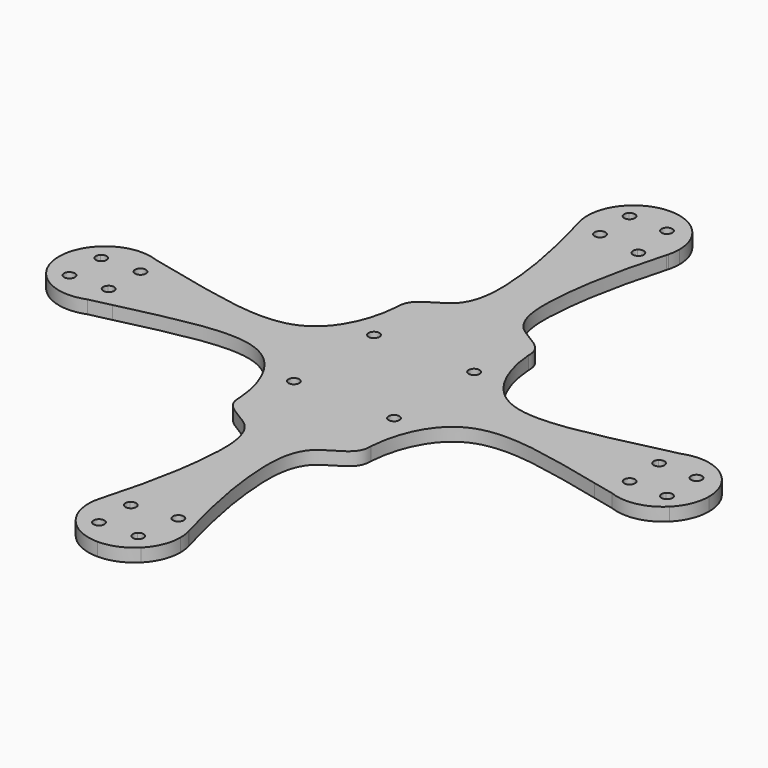
from build123d import *

# Parameters (mm, degrees)
F0_W     = 20
F0_H     = 30
F0_R     = 1.65
F1_DEPTH = 4


with BuildPart() as f1:
    # F0 (on Top) → F1 (new body)
    with BuildSketch(Plane.XY):
        with BuildLine():
            ThreePointArc((9.8994949366, 104.8994949366), (5.3575680531, 107.9343134552), (0, 109))
            Line((0, 109), (0, 95))
            Line((0, 95), (4.4901280605, 99.4901280605))
            ThreePointArc((4.4901280605, 99.4901280605), (4.4901280605, 101.8235804385), (6.8235804385, 101.8235804385))
            Line((6.8235804385, 101.8235804385), (9.8994949366, 104.8994949366))
        make_face()
        with BuildLine():
            Line((0, 95), (0, 109))
            ThreePointArc((0, 109), (-5.3575680531, 107.9343134552), (-9.8994949366, 104.8994949366))
            Line((-9.8994949366, 104.8994949366), (-7.177133829, 102.177133829))
            ThreePointArc((-7.177133829, 102.177133829), (-5.3789799767, 102.5348088687), (-4.3604076401, 101.0104076401))
            ThreePointArc((-4.3604076401, 101.0104076401), (-4.4860064114, 100.3789799767), (-4.8436814511, 99.8436814511))
            Line((-4.8436814511, 99.8436814511), (0, 95))
        make_face()
        with BuildLine():
            Line((6.2578950135, 88.7421049865), (0, 95))
            Line((0, 95), (0, 81))
            ThreePointArc((0, 81), (5.3575680531, 82.0656865448), (9.8994949366, 85.1005050634))
            Line((9.8994949366, 85.1005050634), (8.5913473914, 86.4086526086))
            ThreePointArc((8.5913473914, 86.4086526086), (6.2578950135, 86.4086526086), (6.2578950135, 88.7421049865))
        make_face()
        with BuildLine():
            Line((0, 81), (0, 95))
            Line((0, 95), (-4.4901280605, 90.5098719395))
            ThreePointArc((-4.4901280605, 90.5098719395), (-4.1324530208, 89.9745734139), (-4.0068542495, 89.3431457505))
            ThreePointArc((-4.0068542495, 89.3431457505), (-5.0254265861, 87.8187445219), (-6.8235804385, 88.1764195615))
            Line((-6.8235804385, 88.1764195615), (-9.8994949366, 85.1005050634))
            ThreePointArc((-9.8994949366, 85.1005050634), (-5.3575680531, 82.0656865448), (0, 81))
        make_face()
        with BuildLine():
            Line((-4.4901280605, 90.5098719395), (0, 95))
            Line((0, 95), (-4.8436814511, 99.8436814511))
            ThreePointArc((-4.8436814511, 99.8436814511), (-7.177133829, 99.8436814511), (-7.177133829, 102.177133829))
            Line((-7.177133829, 102.177133829), (-9.8994949366, 104.8994949366))
            ThreePointArc((-9.8994949366, 104.8994949366), (-13.5184120598, 98.6404031894), (-13.5319969205, 91.4104235148))
            add(Edge.make_bspline(
                [(-13.3797592699, 90.8790726917), (-13.4302497753, 91.0559438951), (-13.4809959841, 91.2330606372), (-13.5319969205, 91.4104235148)],
                knots=[0.9938840637, 0.9938840637, 0.9938840637, 0.9938840637, 1, 1, 1, 1], degree=3))
            ThreePointArc((-13.3797592699, 90.8790726917), (-11.9928678831, 87.7770421614), (-9.8994949366, 85.1005050634))
            Line((-9.8994949366, 85.1005050634), (-6.8235804385, 88.1764195615))
            ThreePointArc((-6.8235804385, 88.1764195615), (-6.8235804385, 90.5098719395), (-4.4901280605, 90.5098719395))
        make_face()
        with BuildLine():
            Line((4.4901280605, 99.4901280605), (0, 95))
            Line((0, 95), (6.2578950135, 88.7421049865))
            ThreePointArc((6.2578950135, 88.7421049865), (8.0560488659, 89.0997800262), (9.0746212025, 87.5753787975))
            ThreePointArc((9.0746212025, 87.5753787975), (8.9490224311, 86.9439511341), (8.5913473914, 86.4086526086))
            Line((8.5913473914, 86.4086526086), (9.8994949366, 85.1005050634))
            ThreePointArc((9.8994949366, 85.1005050634), (11.9928678831, 87.7770421614), (13.3797592699, 90.8790726917))
            add(Edge.make_bspline(
                [(13.3797592699, 90.8790726917), (13.4302497753, 91.0559438951), (13.4809959841, 91.2330606372), (13.5319969205, 91.4104235148)],
                knots=[0.9938840637, 0.9938840637, 0.9938840637, 0.9938840637, 1, 1, 1, 1], degree=3))
            ThreePointArc((13.5319969205, 91.4104235148), (13.8825062018, 93.1900216697), (14, 95))
            ThreePointArc((14, 95), (12.9343134552, 100.3575680531), (9.8994949366, 104.8994949366))
            Line((9.8994949366, 104.8994949366), (6.8235804385, 101.8235804385))
            ThreePointArc((6.8235804385, 101.8235804385), (7.1812554781, 101.2882819129), (7.3068542495, 100.6568542495))
            ThreePointArc((7.3068542495, 100.6568542495), (6.2882819129, 99.1324530208), (4.4901280605, 99.4901280605))
        make_face()
        with BuildLine():
            ThreePointArc((9.8994949366, 85.1005050634), (5.3575680531, 82.0656865448), (0, 81))
            Line((0, 81), (0, 30))
            Line((0, 30), (20, 30))
            add(Edge.make_bspline(
                [(20, 30), (20.2946353761, 35.7326359325), (6.8531098255, 37.7432494173), (6.0119172559, 59.8139246806), (9.9463832068, 78.8517548594), (13.3797592699, 90.8790726917)],
                knots=[0, 0, 0, 0, 0.2669632141, 0.5779977645, 0.9938840637, 0.9938840637, 0.9938840637, 0.9938840637], degree=3))
            ThreePointArc((13.3797592699, 90.8790726917), (11.9928678831, 87.7770421614), (9.8994949366, 85.1005050634))
        make_face()
        with BuildLine():
            Line((0, 30), (0, 81))
            ThreePointArc((0, 81), (-5.3575680531, 82.0656865448), (-9.8994949366, 85.1005050634))
            ThreePointArc((-9.8994949366, 85.1005050634), (-11.9928678831, 87.7770421614), (-13.3797592699, 90.8790726917))
            add(Edge.make_bspline(
                [(-20, 30), (-20.2946353761, 35.7326359325), (-6.8531098255, 37.7432494173), (-6.0119172559, 59.8139246806), (-9.9463832068, 78.8517548594), (-13.3797592699, 90.8790726917)],
                knots=[0, 0, 0, 0, 0.2669632141, 0.5779977645, 0.9938840637, 0.9938840637, 0.9938840637, 0.9938840637], degree=3))
            Line((-20, 30), (0, 30))
        make_face()
        with BuildLine():
            add(Edge.make_bspline(
                [(-13.3797592699, 90.8790726917), (-13.4302497753, 91.0559438951), (-13.4809959841, 91.2330606372), (-13.5319969205, 91.4104235148)],
                knots=[0.9938840637, 0.9938840637, 0.9938840637, 0.9938840637, 1, 1, 1, 1], degree=3))
            ThreePointArc((-13.5319969205, 91.4104235148), (-13.4585006125, 91.1439967242), (-13.3797592699, 90.8790726917))
        make_face()
        with Locations((10, 15)):
            Rectangle(F0_W, F0_H)
        with Locations((15.25, 15.25)):
            Circle(F0_R, mode=Mode.SUBTRACT)
        with Locations((-10, 15)):
            Rectangle(F0_W, F0_H)
        with Locations((-15.25, 15.25)):
            Circle(F0_R, mode=Mode.SUBTRACT)
        with BuildLine():
            ThreePointArc((13.3797592699, 90.8790726917), (13.4585006125, 91.1439967242), (13.5319969205, 91.4104235148))
            add(Edge.make_bspline(
                [(13.3797592699, 90.8790726917), (13.4302497753, 91.0559438951), (13.4809959841, 91.2330606372), (13.5319969205, 91.4104235148)],
                knots=[0.9938840637, 0.9938840637, 0.9938840637, 0.9938840637, 1, 1, 1, 1], degree=3))
        make_face()
        with Locations((10, -15)):
            Rectangle(F0_W, F0_H)
        with Locations((15.25, -15.25)):
            Circle(F0_R, mode=Mode.SUBTRACT)
        with Locations((-10, -15)):
            Rectangle(F0_W, F0_H)
        with Locations((-15.25, -15.25)):
            Circle(F0_R, mode=Mode.SUBTRACT)
        with BuildLine():
            add(Edge.make_bspline(
                [(20, 30), (20.6434332622, 21.0878026995), (29.0666934116, 0.5854139886), (55.4305406227, 7.3872741481), (73.4306914551, 11.5693085449)],
                knots=[0, 0, 0, 0, 0.4161099486, 0.9383621207, 0.9383621207, 0.9383621207, 0.9383621207], degree=3))
            Line((20, 30), (20, 0))
            Line((20, 0), (71, 0))
            ThreePointArc((71, 0), (72.0656865448, 5.3575680531), (75.1005050634, 9.8994949366))
            Line((75.1005050634, 9.8994949366), (73.4306914551, 11.5693085449))
        make_face()
        with BuildLine():
            Line((-20, 0), (-20, 30))
            add(Edge.make_bspline(
                [(-20, 30), (-20.6434332622, 21.0878026995), (-29.0666934116, 0.5854139886), (-55.4305406227, 7.3872741481), (-73.4306914551, 11.5693085449)],
                knots=[0, 0, 0, 0, 0.4161099486, 0.9383621207, 0.9383621207, 0.9383621207, 0.9383621207], degree=3))
            Line((-73.4306914551, 11.5693085449), (-75.1005050634, 9.8994949366))
            ThreePointArc((-75.1005050634, 9.8994949366), (-72.0656865448, 5.3575680531), (-71, 0))
            Line((-71, 0), (-20, 0))
        make_face()
        with BuildLine():
            Line((20, -30), (0, -30))
            Line((0, -30), (0, -81))
            ThreePointArc((0, -81), (5.3575680531, -82.0656865448), (9.8994949366, -85.1005050634))
            ThreePointArc((9.8994949366, -85.1005050634), (11.9928678831, -87.7770421614), (13.3797592699, -90.8790726917))
            add(Edge.make_bspline(
                [(20, -30), (20.2946353761, -35.7326359325), (6.8531098255, -37.7432494173), (6.0119172559, -59.8139246806), (9.9463832068, -78.8517548594), (13.3797592699, -90.8790726917)],
                knots=[0, 0, 0, 0, 0.2669632141, 0.5779977645, 0.9938840637, 0.9938840637, 0.9938840637, 0.9938840637], degree=3))
        make_face()
        with BuildLine():
            Line((0, -81), (0, -30))
            Line((0, -30), (-20, -30))
            add(Edge.make_bspline(
                [(-20, -30), (-20.2946353761, -35.7326359325), (-6.8531098255, -37.7432494173), (-6.0119172559, -59.8139246806), (-9.9463832068, -78.8517548594), (-13.3797592699, -90.8790726917)],
                knots=[0, 0, 0, 0, 0.2669632141, 0.5779977645, 0.9938840637, 0.9938840637, 0.9938840637, 0.9938840637], degree=3))
            ThreePointArc((-13.3797592699, -90.8790726917), (-11.9928678831, -87.7770421614), (-9.8994949366, -85.1005050634))
            ThreePointArc((-9.8994949366, -85.1005050634), (-5.3575680531, -82.0656865448), (0, -81))
        make_face()
        with BuildLine():
            Line((-20, -30), (-20, 0))
            Line((-20, 0), (-71, 0))
            ThreePointArc((-71, 0), (-72.0656865448, -5.3575680531), (-75.1005050634, -9.8994949366))
            Line((-75.1005050634, -9.8994949366), (-73.4306914551, -11.5693085449))
            add(Edge.make_bspline(
                [(-20, -30), (-20.6434332622, -21.0878026995), (-29.0666934116, -0.5854139886), (-55.4305406227, -7.3872741481), (-73.4306914551, -11.5693085449)],
                knots=[0, 0, 0, 0, 0.4161099486, 0.9383621207, 0.9383621207, 0.9383621207, 0.9383621207], degree=3))
        make_face()
        with BuildLine():
            Line((71, 0), (20, 0))
            Line((20, 0), (20, -30))
            add(Edge.make_bspline(
                [(20, -30), (20.6434332622, -21.0878026995), (29.0666934116, -0.5854139886), (55.4305406227, -7.3872741481), (73.4306914551, -11.5693085449)],
                knots=[0, 0, 0, 0, 0.4161099486, 0.9383621207, 0.9383621207, 0.9383621207, 0.9383621207], degree=3))
            Line((73.4306914551, -11.5693085449), (75.1005050634, -9.8994949366))
            ThreePointArc((75.1005050634, -9.8994949366), (72.0656865448, -5.3575680531), (71, 0))
        make_face()
        with BuildLine():
            add(Edge.make_bspline(
                [(73.4306914551, 11.5693085449), (75.5551270882, 12.0628856806), (77.7259083603, 12.5619846054), (79.9393690816, 13.0533526233)],
                knots=[0.9383621207, 0.9383621207, 0.9383621207, 0.9383621207, 1, 1, 1, 1], degree=3))
            Line((73.4306914551, 11.5693085449), (75.1005050634, 9.8994949366))
            ThreePointArc((75.1005050634, 9.8994949366), (77.3555218637, 11.7286808305), (79.9393690816, 13.0533526233))
        make_face()
        with BuildLine():
            Line((-75.1005050634, 9.8994949366), (-73.4306914551, 11.5693085449))
            add(Edge.make_bspline(
                [(-73.4306914551, 11.5693085449), (-75.5551270882, 12.0628856806), (-77.7259083603, 12.5619846054), (-79.9393690816, 13.0533526233)],
                knots=[0.9383621207, 0.9383621207, 0.9383621207, 0.9383621207, 1, 1, 1, 1], degree=3))
            ThreePointArc((-79.9393690816, 13.0533526233), (-77.3555218637, 11.7286808305), (-75.1005050634, 9.8994949366))
        make_face()
        with BuildLine():
            ThreePointArc((9.8994949366, -85.1005050634), (5.3575680531, -82.0656865448), (0, -81))
            Line((0, -81), (0, -95))
            Line((0, -95), (6.2578950135, -88.7421049865))
            ThreePointArc((6.2578950135, -88.7421049865), (6.2578950135, -86.4086526086), (8.5913473914, -86.4086526086))
            Line((8.5913473914, -86.4086526086), (9.8994949366, -85.1005050634))
        make_face()
        with BuildLine():
            Line((0, -95), (0, -81))
            ThreePointArc((0, -81), (-5.3575680531, -82.0656865448), (-9.8994949366, -85.1005050634))
            Line((-9.8994949366, -85.1005050634), (-6.8235804385, -88.1764195615))
            ThreePointArc((-6.8235804385, -88.1764195615), (-5.0254265861, -87.8187445219), (-4.0068542495, -89.3431457505))
            ThreePointArc((-4.0068542495, -89.3431457505), (-4.1324530208, -89.9745734139), (-4.4901280605, -90.5098719395))
            Line((-4.4901280605, -90.5098719395), (0, -95))
        make_face()
        with BuildLine():
            ThreePointArc((-75.1005050634, -9.8994949366), (-72.0656865448, -5.3575680531), (-71, 0))
            Line((-71, 0), (-85, 0))
            Line((-85, 0), (-80.5098719395, -4.4901280605))
            ThreePointArc((-80.5098719395, -4.4901280605), (-78.7117180871, -4.1324530208), (-77.6931457505, -5.6568542495))
            ThreePointArc((-77.6931457505, -5.6568542495), (-77.8187445219, -6.2882819129), (-78.1764195615, -6.8235804385))
            Line((-78.1764195615, -6.8235804385), (-75.1005050634, -9.8994949366))
        make_face()
        with BuildLine():
            Line((-85, 0), (-71, 0))
            ThreePointArc((-71, 0), (-72.0656865448, 5.3575680531), (-75.1005050634, 9.8994949366))
            Line((-75.1005050634, 9.8994949366), (-77.822866171, 7.177133829))
            ThreePointArc((-77.822866171, 7.177133829), (-77.4651911313, 6.6418353035), (-77.3395923599, 6.0104076401))
            ThreePointArc((-77.3395923599, 6.0104076401), (-78.3581646965, 4.4860064114), (-80.1563185489, 4.8436814511))
            Line((-80.1563185489, 4.8436814511), (-85, 0))
        make_face()
        with BuildLine():
            ThreePointArc((75.1005050634, 9.8994949366), (72.0656865448, 5.3575680531), (71, 0))
            Line((71, 0), (85, 0))
            Line((85, 0), (80.1563185489, 4.8436814511))
            ThreePointArc((80.1563185489, 4.8436814511), (77.822866171, 4.8436814511), (77.822866171, 7.177133829))
            Line((77.822866171, 7.177133829), (75.1005050634, 9.8994949366))
        make_face()
        with BuildLine():
            Line((85, 0), (71, 0))
            ThreePointArc((71, 0), (72.0656865448, -5.3575680531), (75.1005050634, -9.8994949366))
            Line((75.1005050634, -9.8994949366), (78.1764195615, -6.8235804385))
            ThreePointArc((78.1764195615, -6.8235804385), (78.1764195615, -4.4901280605), (80.5098719395, -4.4901280605))
            Line((80.5098719395, -4.4901280605), (85, 0))
        make_face()
        with BuildLine():
            ThreePointArc((79.9393690816, 13.0533526233), (77.3555218637, 11.7286808305), (75.1005050634, 9.8994949366))
            Line((75.1005050634, 9.8994949366), (77.822866171, 7.177133829))
            ThreePointArc((77.822866171, 7.177133829), (79.6210200233, 7.5348088687), (80.6395923599, 6.0104076401))
            ThreePointArc((80.6395923599, 6.0104076401), (80.5139935886, 5.3789799767), (80.1563185489, 4.8436814511))
            Line((80.1563185489, 4.8436814511), (85, 0))
            Line((85, 0), (89.4901280605, 4.4901280605))
            ThreePointArc((89.4901280605, 4.4901280605), (89.4901280605, 6.8235804385), (91.8235804385, 6.8235804385))
            Line((91.8235804385, 6.8235804385), (94.8994949366, 9.8994949366))
            ThreePointArc((94.8994949366, 9.8994949366), (87.8879674208, 13.6988920784), (79.9393690816, 13.0533526233))
        make_face()
        with BuildLine():
            Line((-77.822866171, 7.177133829), (-75.1005050634, 9.8994949366))
            ThreePointArc((-75.1005050634, 9.8994949366), (-77.3555218637, 11.7286808305), (-79.9393690816, 13.0533526233))
            ThreePointArc((-79.9393690816, 13.0533526233), (-87.8879674208, 13.6988920784), (-94.8994949366, 9.8994949366))
            Line((-94.8994949366, 9.8994949366), (-91.8235804385, 6.8235804385))
            ThreePointArc((-91.8235804385, 6.8235804385), (-90.0254265861, 7.1812554781), (-89.0068542495, 5.6568542495))
            ThreePointArc((-89.0068542495, 5.6568542495), (-89.1324530208, 5.0254265861), (-89.4901280605, 4.4901280605))
            Line((-89.4901280605, 4.4901280605), (-85, 0))
            Line((-85, 0), (-80.1563185489, 4.8436814511))
            ThreePointArc((-80.1563185489, 4.8436814511), (-80.1563185489, 7.177133829), (-77.822866171, 7.177133829))
        make_face()
        with BuildLine():
            Line((4.4901280605, -99.4901280605), (0, -95))
            Line((0, -95), (0, -109))
            ThreePointArc((0, -109), (5.3575680531, -107.9343134552), (9.8994949366, -104.8994949366))
            Line((9.8994949366, -104.8994949366), (6.8235804385, -101.8235804385))
            ThreePointArc((6.8235804385, -101.8235804385), (4.4901280605, -101.8235804385), (4.4901280605, -99.4901280605))
        make_face()
        with BuildLine():
            Line((-4.8436814511, -99.8436814511), (0, -95))
            Line((0, -95), (-4.4901280605, -90.5098719395))
            ThreePointArc((-4.4901280605, -90.5098719395), (-6.8235804385, -90.5098719395), (-6.8235804385, -88.1764195615))
            Line((-6.8235804385, -88.1764195615), (-9.8994949366, -85.1005050634))
            ThreePointArc((-9.8994949366, -85.1005050634), (-11.9928678831, -87.7770421614), (-13.3797592699, -90.8790726917))
            add(Edge.make_bspline(
                [(-13.3797592699, -90.8790726917), (-13.4302497753, -91.0559438951), (-13.4809959841, -91.2330606372), (-13.5319969205, -91.4104235148)],
                knots=[0.9938840637, 0.9938840637, 0.9938840637, 0.9938840637, 1, 1, 1, 1], degree=3))
            ThreePointArc((-13.5319969205, -91.4104235148), (-13.5184120598, -98.6404031894), (-9.8994949366, -104.8994949366))
            Line((-9.8994949366, -104.8994949366), (-7.177133829, -102.177133829))
            ThreePointArc((-7.177133829, -102.177133829), (-7.177133829, -99.8436814511), (-4.8436814511, -99.8436814511))
        make_face()
        with BuildLine():
            Line((6.2578950135, -88.7421049865), (0, -95))
            Line((0, -95), (4.4901280605, -99.4901280605))
            ThreePointArc((4.4901280605, -99.4901280605), (6.2882819129, -99.1324530208), (7.3068542495, -100.6568542495))
            ThreePointArc((7.3068542495, -100.6568542495), (7.1812554781, -101.2882819129), (6.8235804385, -101.8235804385))
            Line((6.8235804385, -101.8235804385), (9.8994949366, -104.8994949366))
            ThreePointArc((9.8994949366, -104.8994949366), (12.9343134552, -100.3575680531), (14, -95))
            ThreePointArc((14, -95), (13.8825062018, -93.1900216697), (13.5319969205, -91.4104235148))
            add(Edge.make_bspline(
                [(13.3797592699, -90.8790726917), (13.4302497753, -91.0559438951), (13.4809959841, -91.2330606372), (13.5319969205, -91.4104235148)],
                knots=[0.9938840637, 0.9938840637, 0.9938840637, 0.9938840637, 1, 1, 1, 1], degree=3))
            ThreePointArc((13.3797592699, -90.8790726917), (11.9928678831, -87.7770421614), (9.8994949366, -85.1005050634))
            Line((9.8994949366, -85.1005050634), (8.5913473914, -86.4086526086))
            ThreePointArc((8.5913473914, -86.4086526086), (8.9490224311, -86.9439511341), (9.0746212025, -87.5753787975))
            ThreePointArc((9.0746212025, -87.5753787975), (8.0560488659, -89.0997800262), (6.2578950135, -88.7421049865))
        make_face()
        with BuildLine():
            Line((0, -109), (0, -95))
            Line((0, -95), (-4.8436814511, -99.8436814511))
            ThreePointArc((-4.8436814511, -99.8436814511), (-4.4860064114, -100.3789799767), (-4.3604076401, -101.0104076401))
            ThreePointArc((-4.3604076401, -101.0104076401), (-5.3789799767, -102.5348088687), (-7.177133829, -102.177133829))
            Line((-7.177133829, -102.177133829), (-9.8994949366, -104.8994949366))
            ThreePointArc((-9.8994949366, -104.8994949366), (-5.3575680531, -107.9343134552), (0, -109))
        make_face()
        with BuildLine():
            ThreePointArc((13.5319969205, -91.4104235148), (13.4585006125, -91.1439967242), (13.3797592699, -90.8790726917))
            add(Edge.make_bspline(
                [(13.3797592699, -90.8790726917), (13.4302497753, -91.0559438951), (13.4809959841, -91.2330606372), (13.5319969205, -91.4104235148)],
                knots=[0.9938840637, 0.9938840637, 0.9938840637, 0.9938840637, 1, 1, 1, 1], degree=3))
        make_face()
        with BuildLine():
            Line((75.1005050634, -9.8994949366), (73.4306914551, -11.5693085449))
            add(Edge.make_bspline(
                [(73.4306914551, -11.5693085449), (75.5551270882, -12.0628856806), (77.7259083603, -12.5619846054), (79.9393690816, -13.0533526233)],
                knots=[0.9383621207, 0.9383621207, 0.9383621207, 0.9383621207, 1, 1, 1, 1], degree=3))
            ThreePointArc((79.9393690816, -13.0533526233), (77.3555218637, -11.7286808305), (75.1005050634, -9.8994949366))
        make_face()
        with BuildLine():
            add(Edge.make_bspline(
                [(-13.3797592699, -90.8790726917), (-13.4302497753, -91.0559438951), (-13.4809959841, -91.2330606372), (-13.5319969205, -91.4104235148)],
                knots=[0.9938840637, 0.9938840637, 0.9938840637, 0.9938840637, 1, 1, 1, 1], degree=3))
            ThreePointArc((-13.3797592699, -90.8790726917), (-13.4585006125, -91.1439967242), (-13.5319969205, -91.4104235148))
        make_face()
        with BuildLine():
            add(Edge.make_bspline(
                [(-73.4306914551, -11.5693085449), (-75.5551270882, -12.0628856806), (-77.7259083603, -12.5619846054), (-79.9393690816, -13.0533526233)],
                knots=[0.9383621207, 0.9383621207, 0.9383621207, 0.9383621207, 1, 1, 1, 1], degree=3))
            Line((-73.4306914551, -11.5693085449), (-75.1005050634, -9.8994949366))
            ThreePointArc((-75.1005050634, -9.8994949366), (-77.3555218637, -11.7286808305), (-79.9393690816, -13.0533526233))
        make_face()
        with BuildLine():
            Line((-89.8436814511, -4.8436814511), (-85, 0))
            Line((-85, 0), (-99, 0))
            ThreePointArc((-99, 0), (-97.9343134552, -5.3575680531), (-94.8994949366, -9.8994949366))
            Line((-94.8994949366, -9.8994949366), (-92.177133829, -7.177133829))
            ThreePointArc((-92.177133829, -7.177133829), (-92.177133829, -4.8436814511), (-89.8436814511, -4.8436814511))
        make_face()
        with BuildLine():
            Line((-80.5098719395, -4.4901280605), (-85, 0))
            Line((-85, 0), (-89.8436814511, -4.8436814511))
            ThreePointArc((-89.8436814511, -4.8436814511), (-89.4860064114, -5.3789799767), (-89.3604076401, -6.0104076401))
            ThreePointArc((-89.3604076401, -6.0104076401), (-90.3789799767, -7.5348088687), (-92.177133829, -7.177133829))
            Line((-92.177133829, -7.177133829), (-94.8994949366, -9.8994949366))
            ThreePointArc((-94.8994949366, -9.8994949366), (-87.8879674208, -13.6988920784), (-79.9393690816, -13.0533526233))
            ThreePointArc((-79.9393690816, -13.0533526233), (-77.3555218637, -11.7286808305), (-75.1005050634, -9.8994949366))
            Line((-75.1005050634, -9.8994949366), (-78.1764195615, -6.8235804385))
            ThreePointArc((-78.1764195615, -6.8235804385), (-80.5098719395, -6.8235804385), (-80.5098719395, -4.4901280605))
        make_face()
        with BuildLine():
            Line((-99, 0), (-85, 0))
            Line((-85, 0), (-89.4901280605, 4.4901280605))
            ThreePointArc((-89.4901280605, 4.4901280605), (-91.8235804385, 4.4901280605), (-91.8235804385, 6.8235804385))
            Line((-91.8235804385, 6.8235804385), (-94.8994949366, 9.8994949366))
            ThreePointArc((-94.8994949366, 9.8994949366), (-97.9343134552, 5.3575680531), (-99, 0))
        make_face()
        with BuildLine():
            Line((89.4901280605, 4.4901280605), (85, 0))
            Line((85, 0), (99, 0))
            ThreePointArc((99, 0), (97.9343134552, 5.3575680531), (94.8994949366, 9.8994949366))
            Line((94.8994949366, 9.8994949366), (91.8235804385, 6.8235804385))
            ThreePointArc((91.8235804385, 6.8235804385), (92.1812554781, 6.2882819129), (92.3068542495, 5.6568542495))
            ThreePointArc((92.3068542495, 5.6568542495), (91.2882819129, 4.1324530208), (89.4901280605, 4.4901280605))
        make_face()
        with BuildLine():
            Line((99, 0), (85, 0))
            Line((85, 0), (89.8436814511, -4.8436814511))
            ThreePointArc((89.8436814511, -4.8436814511), (91.6418353035, -4.4860064114), (92.6604076401, -6.0104076401))
            ThreePointArc((92.6604076401, -6.0104076401), (92.5348088687, -6.6418353035), (92.177133829, -7.177133829))
            Line((92.177133829, -7.177133829), (94.8994949366, -9.8994949366))
            ThreePointArc((94.8994949366, -9.8994949366), (97.9343134552, -5.3575680531), (99, 0))
        make_face()
        with BuildLine():
            Line((89.8436814511, -4.8436814511), (85, 0))
            Line((85, 0), (80.5098719395, -4.4901280605))
            ThreePointArc((80.5098719395, -4.4901280605), (80.8675469792, -5.0254265861), (80.9931457505, -5.6568542495))
            ThreePointArc((80.9931457505, -5.6568542495), (79.9745734139, -7.1812554781), (78.1764195615, -6.8235804385))
            Line((78.1764195615, -6.8235804385), (75.1005050634, -9.8994949366))
            ThreePointArc((75.1005050634, -9.8994949366), (77.3555218637, -11.7286808305), (79.9393690816, -13.0533526233))
            ThreePointArc((79.9393690816, -13.0533526233), (87.8879674208, -13.6988920784), (94.8994949366, -9.8994949366))
            Line((94.8994949366, -9.8994949366), (92.177133829, -7.177133829))
            ThreePointArc((92.177133829, -7.177133829), (89.8436814511, -7.177133829), (89.8436814511, -4.8436814511))
        make_face()
    extrude(amount=F1_DEPTH)


solid = f1.part
